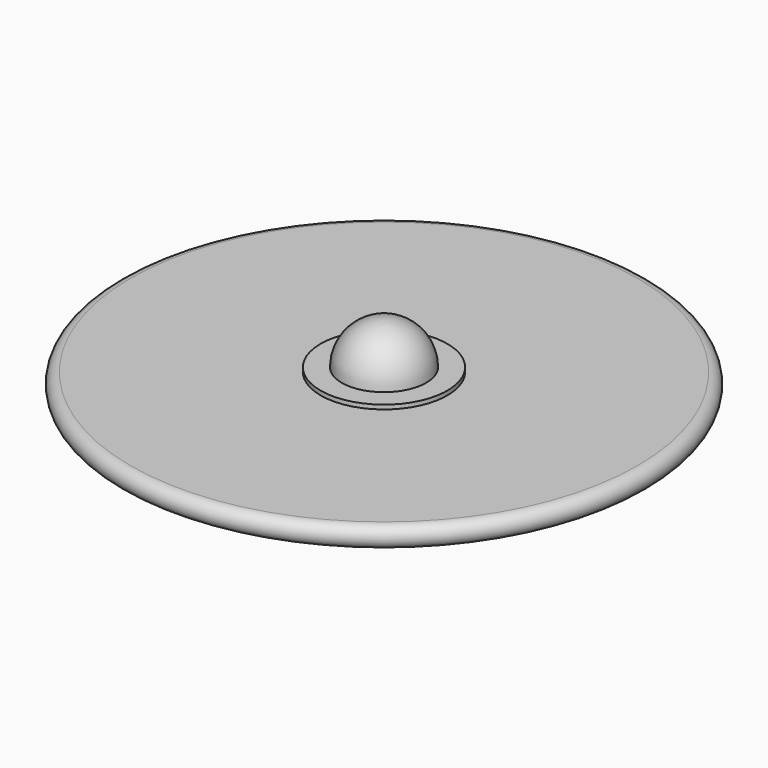
from build123d import *


# Not quite as in the source:
# - ends of sketch curves that miss each other by under 0.0002 mm in the source are joined
# - a feature names something its author has since deleted; it is built from what else it names


with BuildPart() as f1:
    # F0 (on Front) → F1 (revolve)
    with BuildSketch(Plane.XZ):
        with BuildLine():
            Line((0, 2), (-24, 2))
            ThreePointArc((-24, 2), (-25, 1), (-24, 0))
            Line((-24, 0), (0, 0))
            Line((0, 0), (0, 2))
        make_face()
    revolve(axis=Axis((0, 0, 1), (0, 0, -1)))


with BuildPart() as f3:
    # F2 (on Front) → F3 (revolve)
    with BuildSketch(Plane.XZ):
        with BuildLine():
            Line((0, 2.3999979427), (0, 6.4))
            ThreePointArc((0, 6.4), (-2.8284271247, 5.2284250674), (-4, 2.3999979427))
            Line((-4, 2.3999979427), (-5.9987170854, 2.3999979427))
            Line((-5.9987170854, 2.3999979427), (-6, 2))
            Line((-6, 2), (0, 2))
            Line((0, 2), (0, 2.3999979427))
        make_face()
    revolve(axis=Axis((0, 0, 4.3999989713), (0, 0, 1)))


solid = Compound([f1.part, f3.part])
